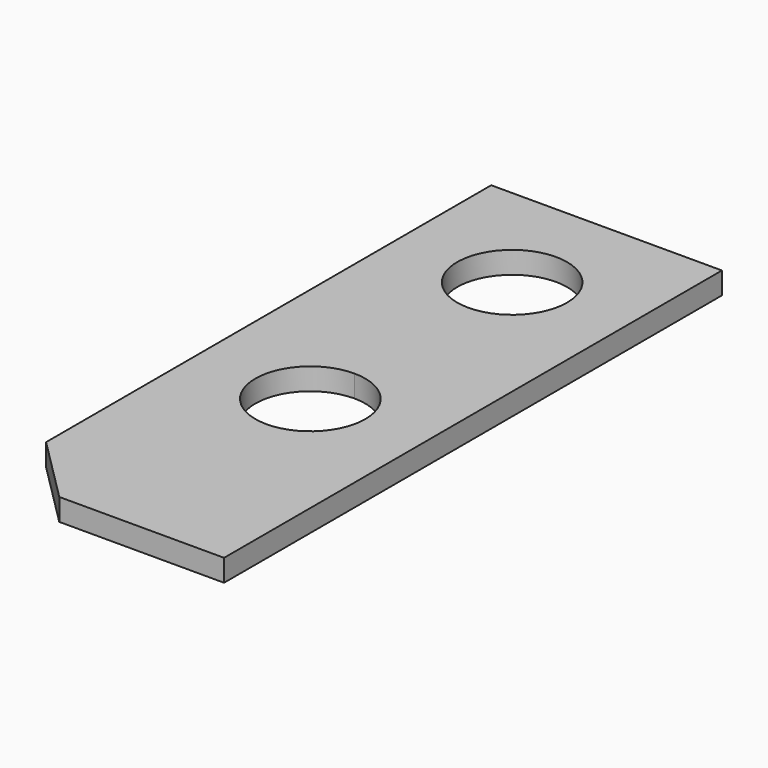
from build123d import *

# Parameters (mm, degrees)
F0_W     = 10.5
F0_H     = 28.32
F1_DEPTH = 1
F3_DEPTH = 1.5
F4_SIZE  = 3


with BuildPart() as f1:
    # F0 (on Top) → F1 (new body)
    with BuildSketch(Plane.XY):
        Rectangle(F0_W, F0_H)
    extrude(amount=F1_DEPTH)

    # F2 (on face) → F3 (cut)
    with BuildSketch(Plane.XY.offset(1)):
        with BuildLine():
            ThreePointArc((2.5, 8.79), (-1.767766953, 10.557766953), (0, 6.29))
            ThreePointArc((0, 6.29), (1.767766953, 7.022233047), (2.5, 8.79))
        make_face()
        with BuildLine():
            ThreePointArc((0, -0.19), (-2.5, -2.69), (0, -5.19))
            ThreePointArc((0, -5.19), (1.767766953, -4.457766953), (2.5, -2.69))
            ThreePointArc((2.5, -2.69), (1.767766953, -0.922233047), (0, -0.19))
        make_face()
    extrude(amount=-F3_DEPTH, mode=Mode.SUBTRACT)

    # F4
    f4_edges = [f1.edges().sort_by_distance(p)[0] for p in [
        (-5.25, -14.16, 0.5),
    ]]
    chamfer(f4_edges, length=F4_SIZE)


solid = f1.part
